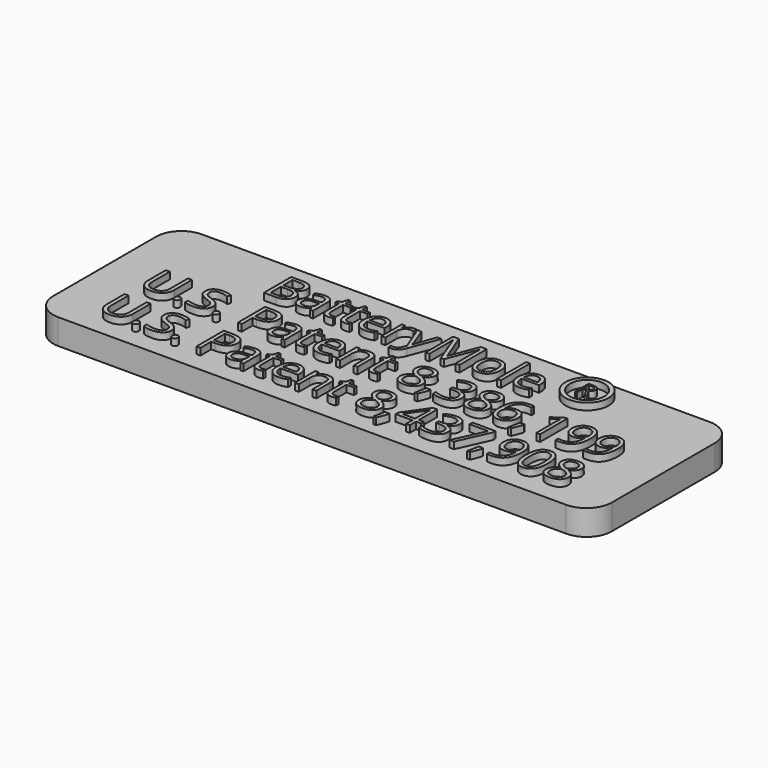
from build123d import *

# Parameters (mm, degrees)
F1_DEPTH       = 1.5
F2_R           = 1.27
F2_R_2         = 1.016
F2_TEXT_SIZE   = 2.8222222222
F2_TEXT_SIZE_2 = 1.4111111111
F3_DEPTH       = 0.4


# Not quite as in the source:
# - Text() gives the source's letters only with a copy of the font that has no kerning and outlines rounded to 1/6400 em; it was checked with that copy


with BuildPart() as f1:
    # F0 (on Top) → F1 (new body)
    with BuildSketch(Plane.XY):
        with BuildLine():
            Line((55.0049993768, 27.1219907546), (25.0049993768, 27.1219907546))
            ThreePointArc((25.0049993768, 27.1219907546), (23.9443392051, 26.6826509263), (23.5049993768, 25.6219907546))
            Line((23.5049993768, 25.6219907546), (23.5049993768, 18.0219907546))
            ThreePointArc((23.5049993768, 18.0219907546), (23.9443392051, 16.9613305828), (25.0049993768, 16.5219907546))
            Line((25.0049993768, 16.5219907546), (55.0049993768, 16.5219907546))
            ThreePointArc((55.0049993768, 16.5219907546), (56.0656595486, 16.9613305828), (56.5049993768, 18.0219907546))
            Line((56.5049993768, 18.0219907546), (56.5049993768, 25.6219907546))
            ThreePointArc((56.5049993768, 25.6219907546), (56.0656595486, 26.6826509263), (55.0049993768, 27.1219907546))
        make_face()
    extrude(amount=F1_DEPTH)

    # F2 (on face) → F3 (join)
    with BuildSketch(Plane.XY.offset(1.5)):
        with Locations((49.0754842758, 25.4774056375)):
            Circle(F2_R)
        with Locations((49.0754842758, 25.4774056375)):
            Circle(F2_R_2, mode=Mode.SUBTRACT)
        with Locations((31.0906629519, 23.7570720532)):
            Text('BatteryMole', F2_TEXT_SIZE, font='Open Sans', text_align=(TextAlign.LEFT, TextAlign.BOTTOM))
        with Locations((26.1723455042, 20.6714986019)):
            Text('U.S. Patent 8,386,199', F2_TEXT_SIZE, font='Open Sans', text_align=(TextAlign.LEFT, TextAlign.BOTTOM))
        with Locations((26.1723436415, 17.6242483907)):
            Text('U.S. Patent 8,437,908', F2_TEXT_SIZE, font='Open Sans', text_align=(TextAlign.LEFT, TextAlign.BOTTOM))
        with Locations((48.600114882, 25.0047299143)):
            Text('R', F2_TEXT_SIZE_2, font='Open Sans', text_align=(TextAlign.LEFT, TextAlign.BOTTOM))
    extrude(amount=F3_DEPTH)


solid = f1.part
